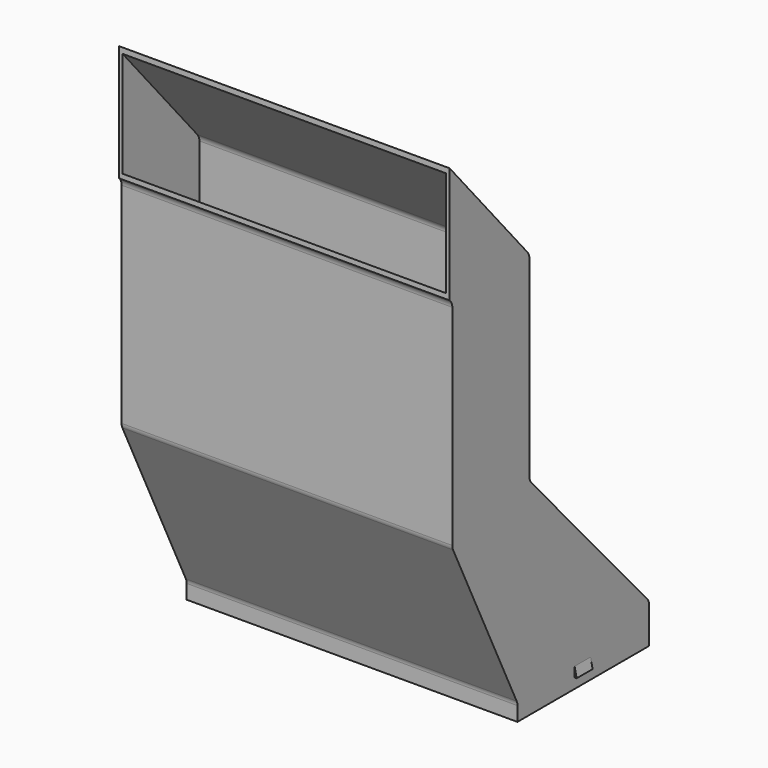
from build123d import *

# Parameters (mm, degrees)
F1_DEPTH    = 99.5
F2_T        = -1.1
F3_R        = 3
F4_W        = 6
F4_H        = 3
F5_DEPTH    = 1
F6_T4_DEPTH = 31.981320863
F7_W        = 6
F7_H        = 3
F8_DEPTH    = 1
F9_T4_DEPTH = 31.981320863


# Not quite as in the source:
# - a fillet or chamfer that OpenCascade refuses, or shapes differently, is made with other operations: its cross-section is extruded or revolved along the edge and cut away or added


with BuildPart() as f1:
    # F0 (on Right) → F1 (new body)
    with BuildSketch(Plane.YZ):
        Polygon((-49.5, 0), (0, 0), (0, 12), (-45, 62), (-45, 122), (-75, 157), (-75, 122), (-74, 121), (-74, 56), (-49.5, 5), align=None)
    extrude(amount=F1_DEPTH)

    # F2
    f2_openings = [f1.faces().sort_by_distance(p)[0] for p in [
        (49.75, -75, 139.5),
        (49.75, -24.75, 0),
    ]]
    offset(amount=F2_T, openings=f2_openings, kind=Kind.INTERSECTION)

    # F3
    f3_edges = [f1.edges().sort_by_distance(p)[0] for p in [
        (49.75, -74, 121),
        (49.75, -74, 56),
        (49.75, -49.5, 5),
        (49.75, 0, 12),
        (49.75, -45, 62),
        (49.75, -45, 122),
        (49.75, -1.1, 11.57789),
        (49.75, -46.1, 61.57789),
        (49.75, -72.9, 56.250512),
        (49.75, -46.1, 121.593084),
        (49.75, -72.9, 121.455635),
        (49.75, -48.4, 5.250512),
    ]]
    fillet(f3_edges, radius=F3_R)

    # F4 (on face) → F5 (join)
    with BuildSketch(Plane(origin=(0, 0, 0), x_dir=(0, -1, 0), z_dir=(-1, 0, 0))):
        with Locations((25, 4.5)):
            Rectangle(F4_W, F4_H)
    extrude(amount=F5_DEPTH)

    # F6: chamfer of 1 x 5 on 1 edges, made by hand


with BuildPart() as f6_tool2:
    # F6_s3 → F6_t4 (new body)
    with BuildSketch(Plane.XZ.offset(40.9906604315)):
        Polygon((0, 6), (-1, 1), (-1, 6), align=None)
    extrude(amount=-F6_T4_DEPTH)

    split(bisect_by=Plane.YZ, keep=Keep.BOTTOM)


with BuildPart() as f1_1:
    add(f1.part)

    # F6_t1: cut F6_tool2
    add(f6_tool2.part, mode=Mode.SUBTRACT)

    # F7 (on face) → F8 (join)
    with BuildSketch(Plane.YZ.offset(99.5)):
        with Locations((-25, 4.5)):
            Rectangle(F7_W, F7_H)
    extrude(amount=F8_DEPTH)

    # F9: chamfer of 1 x 5 on 1 edges, made by hand


with BuildPart() as f9_tool2:
    # F9_s3 → F9_t4 (new body)
    with BuildSketch(Plane.XZ.offset(9.0093395685)):
        Polygon((99.5, 6), (100.5, 1), (100.5, 6), align=None)
    extrude(amount=F9_T4_DEPTH)

    split(bisect_by=Plane.YZ.offset(99.5), keep=Keep.TOP)


with BuildPart() as f1_2:
    add(f1_1.part)

    # F9_t1: cut F9_tool2
    add(f9_tool2.part, mode=Mode.SUBTRACT)


solid = f1_2.part
